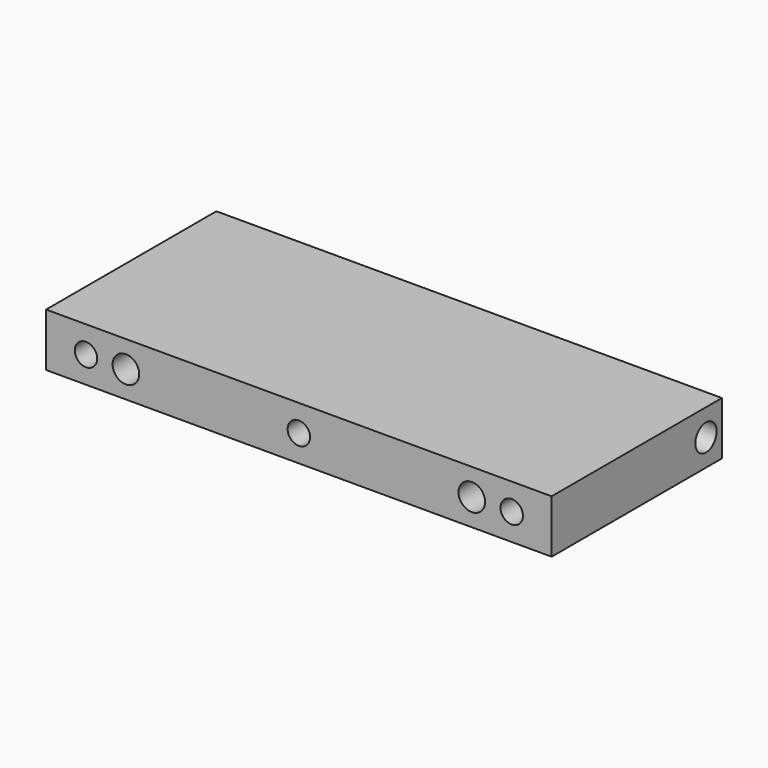
from build123d import *

# Parameters (mm, degrees)
F0_W     = 241.3
F0_H     = 25.4
F1_DEPTH = 50.8
F2_R     = 6.35
F3_DEPTH = 24.765
F5_D     = 7.9375
F5_DEPTH = 27.0002
F5_TIP   = 2.3846655818
F7_D     = 10.71626
F7_DEPTH = 35.179
F7_TIP   = 3.2194893086
F8_D     = 12.7
F8_DEPTH = 38.1
F8_TIP   = 3.8154649308


# Not quite as in the source:
# - a length typed as a fraction of an inch, garbled in the dataset ("3 / 203.2 mm" for 3/8 in), is restored


with BuildPart() as f1:
    # F0 (on Front) → F1 (new body, symmetric)
    with BuildSketch(Plane.XZ):
        Rectangle(F0_W, F0_H)
    extrude(amount=F1_DEPTH, both=True)

    # F2 (on face) → F3 (cut)
    with BuildSketch(Plane.YZ.offset(120.65)):
        with Locations((41.275, 0)):
            Circle(F2_R)
    extrude(amount=-F3_DEPTH, mode=Mode.SUBTRACT)

    # F5
    with Locations(Plane.YZ.offset(95.885)):
        with Locations((41.275, 0)):
            Hole(F5_D / 2, depth=F5_DEPTH)
            with Locations((0, 0, -(F5_DEPTH + F5_TIP / 2))):  # 118° drill point
                Cone(0, F5_D / 2, F5_TIP, mode=Mode.SUBTRACT)

    # F7
    with Locations(Plane.XZ.offset(50.8)):
        with Locations((-101.6, 0), (0, 0), (101.6, 0)):
            Hole(F7_D / 2, depth=F7_DEPTH)
            with Locations((0, 0, -(F7_DEPTH + F7_TIP / 2))):  # 118° drill point
                Cone(0, F7_D / 2, F7_TIP, mode=Mode.SUBTRACT)

    # F8
    with Locations(Plane.XZ.offset(50.8)):
        with Locations((-82.55, 0), (82.55, 0)):
            Hole(F8_D / 2, depth=F8_DEPTH)
            with Locations((0, 0, -(F8_DEPTH + F8_TIP / 2))):  # 118° drill point
                Cone(0, F8_D / 2, F8_TIP, mode=Mode.SUBTRACT)


solid = f1.part
